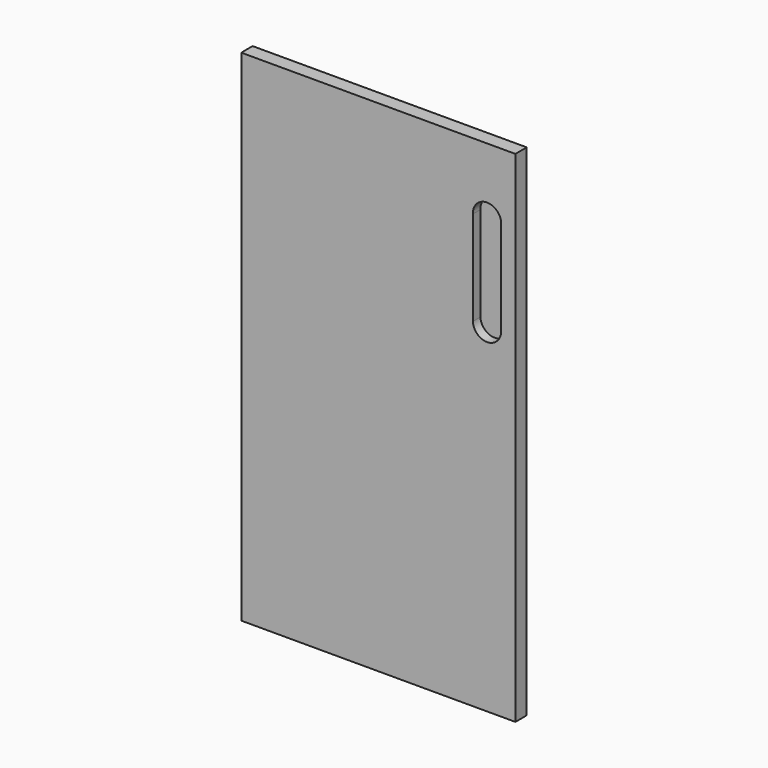
from build123d import *

# Parameters (mm, degrees)
F0_W     = 290
F0_H     = 529
F1_DEPTH = 15
F3_DEPTH = 10


with BuildPart() as f1:
    # F0 (on Front) → F1 (new body)
    with BuildSketch(Plane.XZ):
        with Locations((145, -264.5)):
            Rectangle(F0_W, F0_H)
    extrude(amount=F1_DEPTH)

    # F2 (on face) → F3 (cut)
    with BuildSketch(Plane.XZ.offset(15)):
        with BuildLine():
            Line((245.0136655844, -169.3598587771), (245.0136655844, -170.6401412229))
            ThreePointArc((245.0136655844, -170.6401412229), (260.3201435355, -184.9965832147), (275, -170))
            ThreePointArc((275, -170), (260.3201435355, -155.0034167853), (245.0136655844, -169.3598587771))
        make_face()
        with BuildLine():
            ThreePointArc((245.0136655844, -169.3598587771), (260.3201435355, -155.0034167853), (275, -170))
            Line((275.0000000457, -170), (274.9922312187, -70.4827039319))
            ThreePointArc((274.9922312187, -70.4827039319), (260.0787738422, -84.9997931546), (245.0136655844, -70.6401412229))
            Line((245.0136655844, -70.6401412229), (245.0136655844, -169.3598587771))
        make_face()
        with BuildLine():
            ThreePointArc((245.0136655844, -70.6401412229), (260.0787738422, -84.9997931546), (274.9922312187, -70.4827039319))
            Line((274.9922312187, -70.4827039319), (274.9921556713, -69.5149553341))
            ThreePointArc((274.9921556713, -69.5149553341), (259.4373995265, -55.0105543562), (245.0136655844, -70.6401412229))
        make_face()
    extrude(amount=-F3_DEPTH, mode=Mode.SUBTRACT)


solid = f1.part
